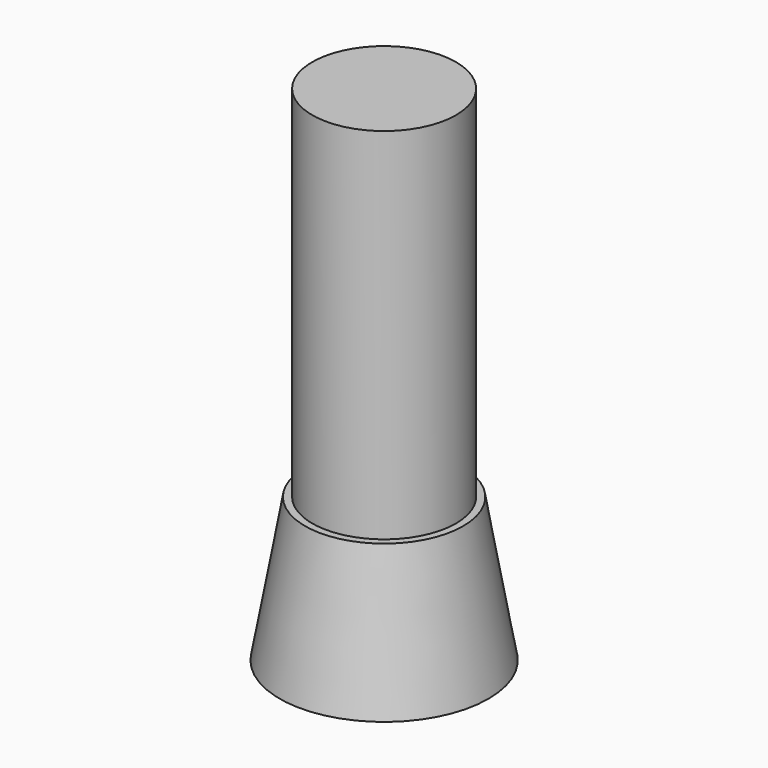
from build123d import *

# Parameters (mm, degrees)
F0_R     = 12.7
F1_DEPTH = 88.9
F0_R_2   = 19.05
F2_DEPTH = 25.4


# Not quite as in the source:
# - a fillet or chamfer that OpenCascade refuses, or shapes differently, is made with other operations: its cross-section is extruded or revolved along the edge and cut away or added


with BuildPart() as f1:
    # F0 (on Top) → F1 (new body)
    with BuildSketch(Plane.XY):
        Circle(F0_R)
    extrude(amount=F1_DEPTH)

    # F0 (on Top) → F2 (join)
    with BuildSketch(Plane.XY):
        Circle(F0_R_2)
        Circle(F0_R, mode=Mode.SUBTRACT)
    extrude(amount=F2_DEPTH)

    # F3: chamfer of 5.08 x 28.8101116437 on 1 edges, made by hand

    # F3_s1 → F3_t2 (revolve, cut)
    with BuildSketch(Plane.XZ):
        Polygon((13.97, 25.4), (19.05, -3.4101116437), (19.05, 25.4), align=None)
    revolve(axis=Axis((0, 0, 25.4), (0, 0, 1)), mode=Mode.SUBTRACT)


solid = f1.part
